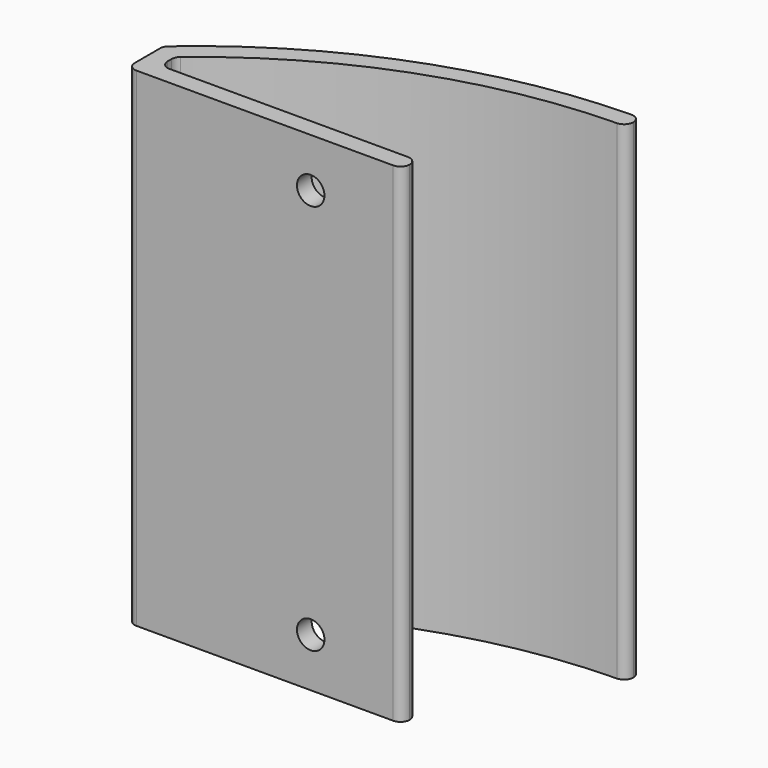
from build123d import *

# Parameters (mm, degrees)
F1_DEPTH = 80
F2_R     = 2.25
F3_DEPTH = 3
F4_R     = 1.49999


# Not quite as in the source:
# - a fillet or chamfer is up to 0.001 mm smaller than in the source, because OpenCascade refuses the exact size
# - a feature names something its author has since deleted; it is built from what else it names


with BuildPart() as f1:
    # F0 (on Top) → F1 (new body)
    with BuildSketch(Plane.XY):
        with BuildLine():
            Line((45, 3), (3, 3))
            Line((3, 3), (3, 6))
            ThreePointArc((3, 6), (29.6273152762, 21.5830013932), (60, 27))
            Line((60, 27), (60, 30))
            ThreePointArc((60, 30), (27.9372056463, 24.1546059211), (0, 7.3705672421))
            Line((0, 7.3705672421), (0, 0))
            Line((0, 0), (45, 0))
            Line((45, 0), (45, 3))
        make_face()
    extrude(amount=F1_DEPTH)

    # F2 (on face) → F3 (cut, through all)
    with BuildSketch(Plane.XZ):
        with Locations((30, 72)):
            Circle(F2_R)
        with Locations((30, 8)):
            Circle(F2_R)
    extrude(amount=-F3_DEPTH, mode=Mode.SUBTRACT)

    # F4 (radius 1.5 in the source; OpenCascade refuses exactly that, so slightly less here)
    f4_edges = [f1.edges().sort_by_distance(p)[0] for p in [
        (45, 0, 40),
        (45, 3, 40),
        (0, 0, 40),
        (0, 7.370567, 40),
        (60, 30, 40),
        (60, 27, 40),
        (3, 3, 40),
        (3, 6, 40),
    ]]
    fillet(f4_edges, radius=F4_R)


solid = f1.part
